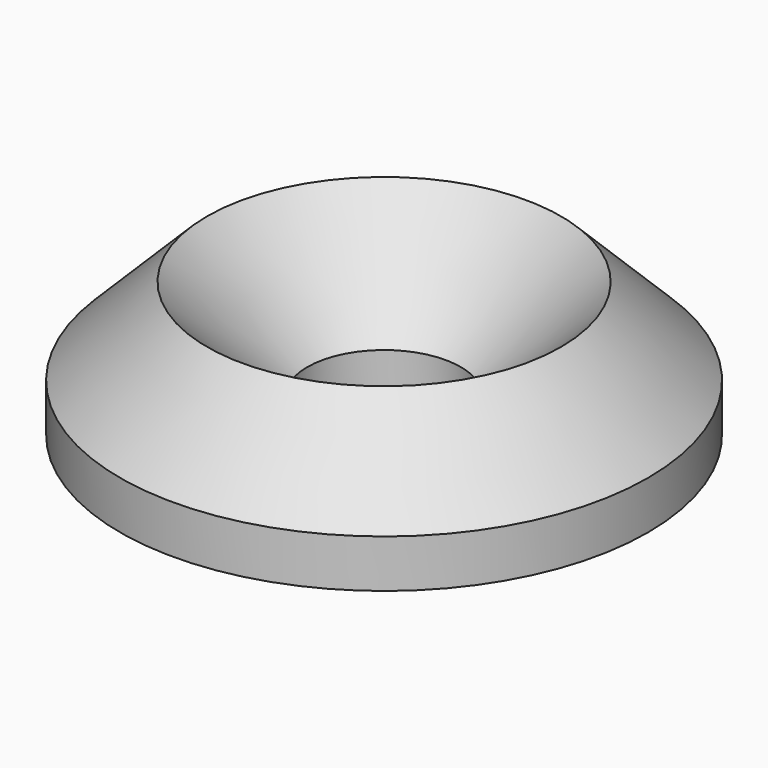
from build123d import *

# Parameters (mm, degrees)
F0_R           = 5.5
F1_DEPTH       = 3
F3_D           = 3.2
F3_DEPTH       = 12
F3_CSINK_D     = 7.75
F3_CSINK_ANGLE = 90
F3_TIP         = 0.9613769904


# Not quite as in the source:
# - a fillet or chamfer that OpenCascade refuses, or shapes differently, is made with other operations: its cross-section is extruded or revolved along the edge and cut away or added


with BuildPart() as f1:
    # F0 (on Top) → F1 (new body)
    with BuildSketch(Plane.XY):
        with Locations((-42.9622493684, 14.7040970623)):
            Circle(F0_R)
    extrude(amount=F1_DEPTH)

    # F3
    with Locations(Plane.XY.offset(3)):
        with Locations((-42.9622493684, 14.7040970623)):
            CounterSinkHole(F3_D / 2, F3_CSINK_D / 2, depth=F3_DEPTH, counter_sink_angle=F3_CSINK_ANGLE)
            with Locations((0, 0, -(F3_DEPTH + F3_TIP / 2))):  # 118° drill point
                Cone(0, F3_D / 2, F3_TIP, mode=Mode.SUBTRACT)

    # F4: chamfer of 2 on 1 edges, made by hand

    # F4_s1 → F4_t2 (revolve, cut)
    with BuildSketch(Plane.XZ.offset(-14.7040970623)):
        Polygon((-37.4622493684, 1), (-39.4622493684, 3), (-37.4622493684, 3), align=None)
    revolve(axis=Axis((-42.9622493684, 14.7040970623, 3), (0, 0, 1)), mode=Mode.SUBTRACT)


solid = f1.part
